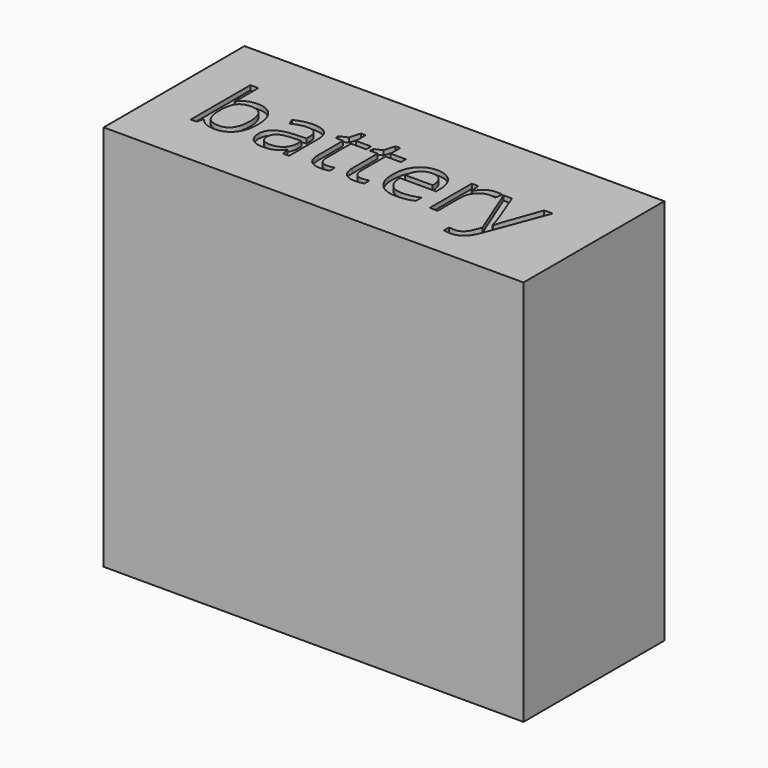
from build123d import *

# Parameters (mm, degrees)
F0_W         = 181.102
F0_H         = 75.946
F1_DEPTH     = 166.878
F2_TEXT_SIZE = 42.3333333333
F3_DEPTH     = 2


# Not quite as in the source:
# - Text() gives the source's letters only with a copy of the font that has no kerning and outlines rounded to 1/6400 em; it was checked with that copy


with BuildPart() as f1:
    # F0 (on Top) → F1 (new body)
    with BuildSketch(Plane.XY):
        Rectangle(F0_W, F0_H)
    extrude(amount=F1_DEPTH)

    # F2 (on face) → F3 (cut)
    with BuildSketch(Plane.XY.offset(166.878)):
        with Locations((-74.8663055682, -15.2004890102)):
            Text('battery', F2_TEXT_SIZE, font='Open Sans', text_align=(TextAlign.LEFT, TextAlign.BOTTOM))
    extrude(amount=-F3_DEPTH, mode=Mode.SUBTRACT)


solid = f1.part
